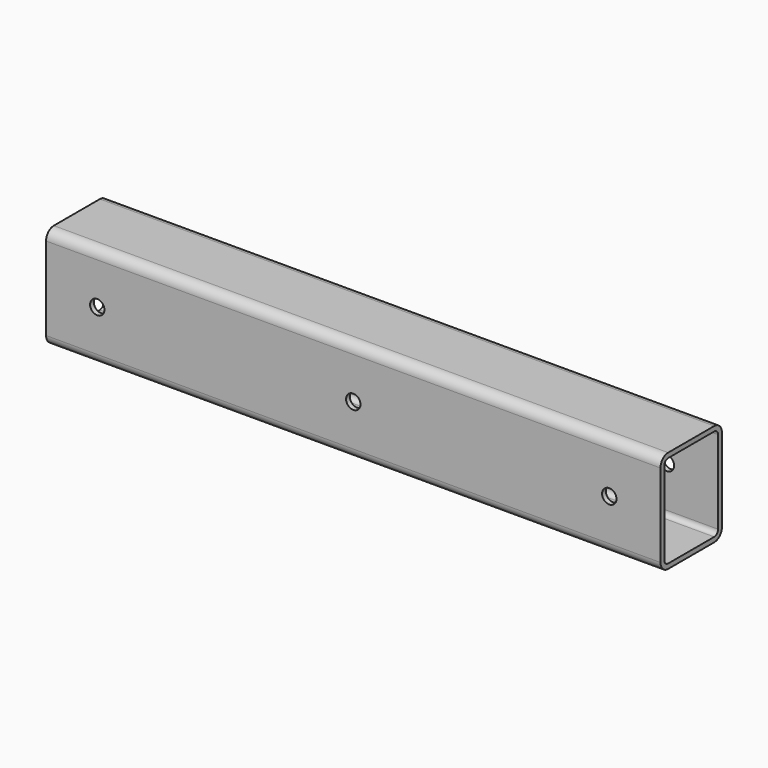
from build123d import *

# Parameters (mm, degrees)
F2_DEPTH = 304.8
F4_D     = 14.2875


# Not quite as in the source:
# - a variable given as a bare number and used for a length is read in inches; the dataset says mm whatever the document's units were


with BuildPart() as f2:
    # F1 (on Right) → F2 (new body, symmetric)
    with BuildSketch(Plane.YZ):
        with BuildLine():
            Line((28.575, 50.8), (-28.575, 50.8))
            ThreePointArc((-28.575, 50.8), (-35.3101920908, 48.0101920908), (-38.1, 41.275))
            Line((-38.1, 41.275), (-38.1, -41.275))
            ThreePointArc((-38.1, -41.275), (-35.3101920908, -48.0101920908), (-28.575, -50.8))
            Line((-28.575, -50.8), (28.575, -50.8))
            ThreePointArc((28.575, -50.8), (35.3101920908, -48.0101920908), (38.1, -41.275))
            Line((38.1, -41.275), (38.1, 41.275))
            ThreePointArc((38.1, 41.275), (35.3101920908, 48.0101920908), (28.575, 50.8))
        make_face()
        with BuildLine():
            ThreePointArc((-33.3375, 41.275), (-31.9425960454, 44.6425960454), (-28.575, 46.0375))
            Line((-28.575, 46.0375), (28.575, 46.0375))
            ThreePointArc((28.575, 46.0375), (31.9425960454, 44.6425960454), (33.3375, 41.275))
            Line((33.3375, 41.275), (33.3375, -41.275))
            ThreePointArc((33.3375, -41.275), (31.9425960454, -44.6425960454), (28.575, -46.0375))
            Line((28.575, -46.0375), (-28.575, -46.0375))
            ThreePointArc((-28.575, -46.0375), (-31.9425960454, -44.6425960454), (-33.3375, -41.275))
            Line((-33.3375, -41.275), (-33.3375, 41.275))
        make_face(mode=Mode.SUBTRACT)
    extrude(amount=F2_DEPTH, both=True)

    # F4 (through all)
    with Locations(Plane.XZ.offset(38.1)):
        with Locations((-254, 0), (0, 0), (254, 0)):
            Hole(F4_D / 2)


solid = f2.part
